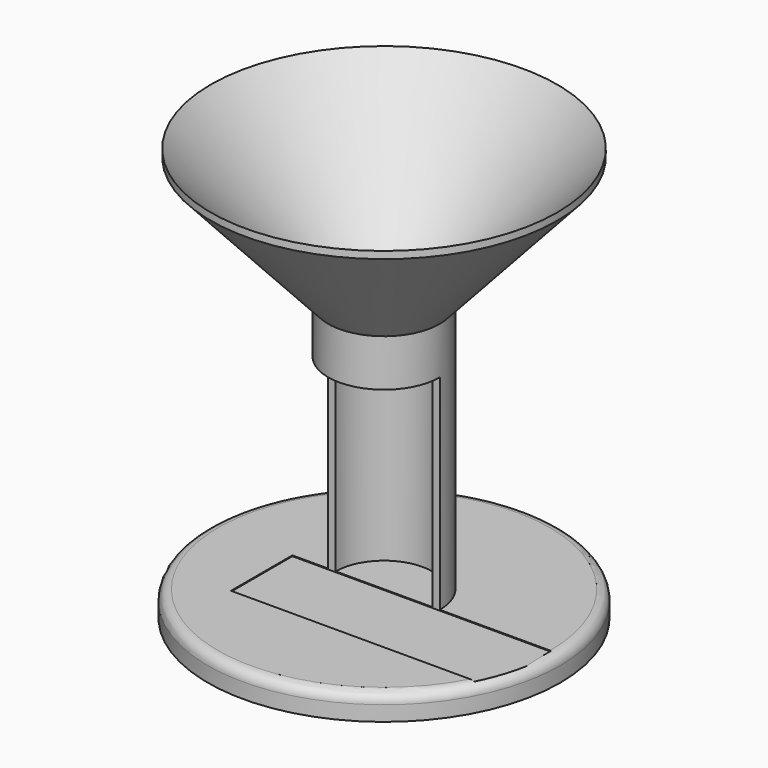
from build123d import *

# Parameters (mm, degrees)
F2_W        = 38.7379527092
F2_H        = 101.6
F2_H_2      = 2.0811606664
F3_DEPTH    = 65.278
F4_T2_ANGLE = 342.3977360444
F4_T4_ANGLE = 26.640456748


# Not quite as in the source:
# - a fillet or chamfer that OpenCascade refuses, or shapes differently, is made with other operations: its cross-section is extruded or revolved along the edge and cut away or added
# - a feature names something its author has since deleted; it is built from what else it names


with BuildPart() as f1:
    # F0 (on Front) → F1 (revolve)
    with BuildSketch(Plane.XZ):
        Polygon((-19.05, -101.1886583478), (-19.05, -113.8886583478), (69.85, -113.8886583478), (69.85, -101.1886583478), (9.1183487131, -101.1886583478), (5.3083487131, -101.1886583478), align=None)
        Polygon((5.3083487131, 21.6246411156), (5.3083487131, -101.1886583478), (9.1183487131, -101.1886583478), (9.1183487131, 25.8113416522), align=None)
        Polygon((0, 15.7914478332), (5.3083487131, 21.6246411156), (9.1183487131, 25.8113416522), (68.3819557915, 90.9344323502), (68.3744283423, 94.5670089535), (-0.0075274492, 19.4240244364), (-11.8764168927, 6.3816397113), (-12.0276177274, 2.5746411156), align=None)
    revolve(axis=Axis((-19.05, 0, -107.5386583478), (0, 0, 1)))

    # F2 (on Right) → F3 (cut, symmetric)
    with BuildSketch(Plane.YZ):
        with Locations((-19.3689763546, -50.8)):
            Rectangle(F2_W, F2_H)
        with Locations((-19.3689763546, 1.0405803332)):
            Rectangle(F2_W, F2_H_2)
    extrude(amount=F3_DEPTH, both=True, mode=Mode.SUBTRACT)

    # F4: fillet of radius 5.08 on 1 edges, made by hand

    # F4_s1 → F4_t2 (revolve, cut)
    with BuildSketch(Plane.XZ):
        with BuildLine():
            ThreePointArc((69.85, -106.2686583478), (68.3621024484, -102.6765558993), (64.77, -101.1886583478))
            Line((64.77, -101.1886583478), (69.85, -101.1886583478))
            Line((69.85, -101.1886583478), (69.85, -106.2686583478))
        make_face()
    revolve(axis=Axis((-19.05, 0, -101.1886583478), (0, 0, 1)), revolution_arc=F4_T2_ANGLE, mode=Mode.SUBTRACT)

    # F4_s3 → F4_t4 (revolve, cut)
    with BuildSketch(Plane(origin=(-3.8300767646, -7.635016329, 0), x_dir=(0, 0, 1), z_dir=(-0.4483903416, -0.8938378497, 0))):
        with BuildLine():
            ThreePointArc((-106.2686583478, -71.8723889628), (-102.6765558993, -70.3844914112), (-101.1886583478, -66.7923889628))
            Line((-101.1886583478, -66.7923889628), (-101.1886583478, -71.8723889628))
            Line((-101.1886583478, -71.8723889628), (-106.2686583478, -71.8723889628))
        make_face()
    revolve(axis=Axis((-19.05, 0, -101.1886583478), (0, 0, 1)), revolution_arc=F4_T4_ANGLE, mode=Mode.SUBTRACT)


solid = f1.part
